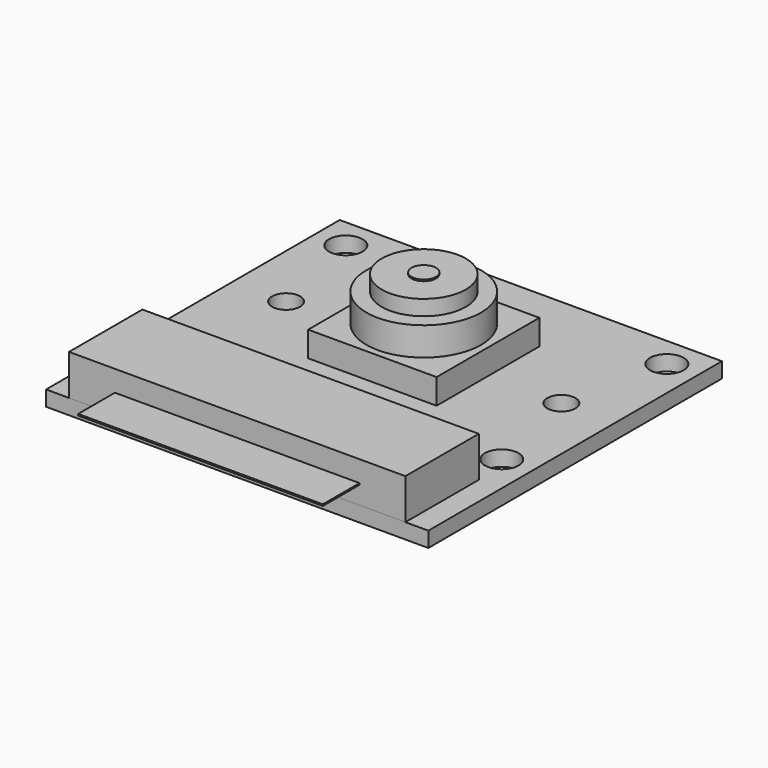
from build123d import *

# Parameters (mm, degrees)
F0_W      = 25
F0_H      = 24
F0_R      = 1.1
F1_DEPTH  = 1
F2_R      = 0.92
F3_DEPTH  = 1
F2_W      = 8.4
F2_H      = 8.4
F2_R_2    = 3.75
F2_R_3    = 2.75
F4_DEPTH  = 1.65
F5_DEPTH  = 3.51
F6_DEPTH  = 4.51
F7_R      = 0.8
F8_DEPTH  = 0.1
F9_W      = 22
F9_H      = 6
F10_DEPTH = 2.65
F12_W     = 16
F12_H     = 3
F13_DEPTH = 0.1


with BuildPart() as f1:
    # F0 (on Top) → F1 (new body)
    with BuildSketch(Plane.XY):
        Rectangle(F0_W, F0_H)
        with Locations((-10.5, -3.5)):
            Circle(F0_R, mode=Mode.SUBTRACT)
        with Locations((10.5, -3.5)):
            Circle(F0_R, mode=Mode.SUBTRACT)
        with Locations((-10.5, 10)):
            Circle(F0_R, mode=Mode.SUBTRACT)
        with Locations((10.5, 10)):
            Circle(F0_R, mode=Mode.SUBTRACT)
    extrude(amount=F1_DEPTH)

    # F2 (on face) → F3 (cut, through all)
    with BuildSketch(Plane.XY.offset(1)):
        with Locations((-9, 3.25)):
            Circle(F2_R)
        with Locations((9, 3.25)):
            Circle(F2_R)
    extrude(amount=-F3_DEPTH, mode=Mode.SUBTRACT)


with BuildPart() as f4:
    # F2 (on face) → F4 (new body)
    with BuildSketch(Plane.XY.offset(1)):
        with Locations((0, 3.25)):
            Rectangle(F2_W, F2_H)
        with Locations((0, 3.25)):
            Circle(F2_R_2, mode=Mode.SUBTRACT)
        with Locations((0, 3.25)):
            Circle(F2_R_2)
        with Locations((0, 3.25)):
            Circle(F2_R_3, mode=Mode.SUBTRACT)
        with Locations((0, 3.25)):
            Circle(F2_R_3)
    extrude(amount=F4_DEPTH)

    # F2 (on face) → F5 (join)
    with BuildSketch(Plane.XY.offset(1)):
        with Locations((0, 3.25)):
            Circle(F2_R_2)
        with Locations((0, 3.25)):
            Circle(F2_R_3, mode=Mode.SUBTRACT)
        with Locations((0, 3.25)):
            Circle(F2_R_3)
    extrude(amount=F5_DEPTH)

    # F2 (on face) → F6 (join)
    with BuildSketch(Plane.XY.offset(1)):
        with Locations((0, 3.25)):
            Circle(F2_R_3)
    extrude(amount=F6_DEPTH)


with BuildPart() as f8:
    # F7 (on face) → F8 (new body)
    with BuildSketch(Plane.XY.offset(5.51)):
        with Locations((0, 3.25)):
            Circle(F7_R)
    extrude(amount=F8_DEPTH)


with BuildPart() as f10:
    # F9 (on face) → F10 (new body)
    with BuildSketch(Plane.XY.offset(1)):
        with Locations((0, -9)):
            Rectangle(F9_W, F9_H)
    extrude(amount=F10_DEPTH)


with BuildPart() as f13:
    # F12 (on offset) → F13 (new body)
    with BuildSketch(Plane(origin=(0, 0, 2.275), x_dir=(1, 0, 0), z_dir=(0, 0, -1))):
        with Locations((0, 13.5)):
            Rectangle(F12_W, F12_H)
    extrude(amount=F13_DEPTH)


solid = Compound([f1.part, f4.part, f8.part, f10.part, f13.part])
